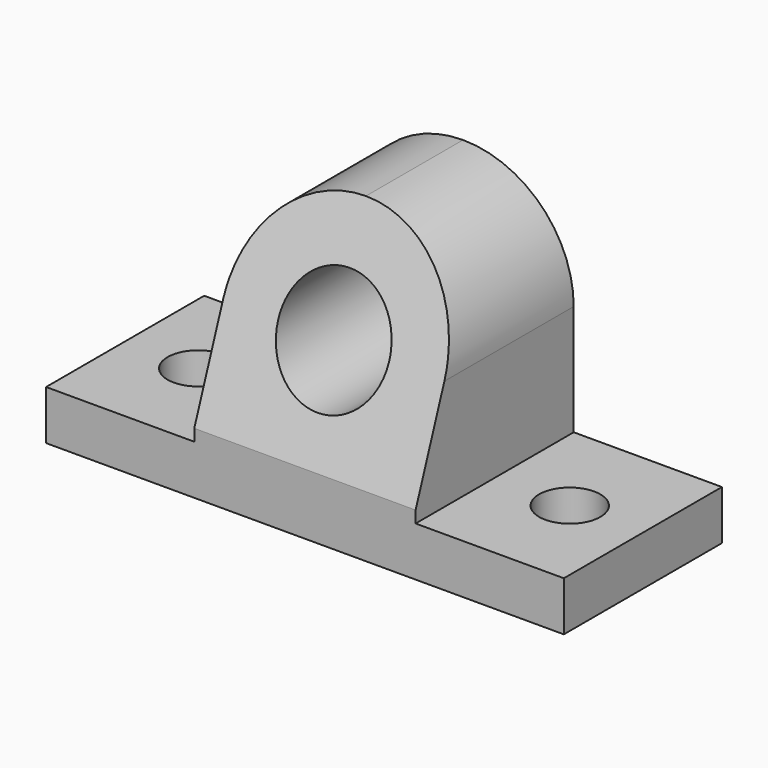
from build123d import *

# Parameters (mm, degrees)
F0_W     = 50.8
F0_H     = 12.7
F0_H_2   = 3.048
F1_DEPTH = 56.896
F2_DEPTH = 94.996
F3_DEPTH = 38.1
F4_R     = 28.44799
F6_DEPTH = 51.054
F8_DEPTH = 42.418


# Not quite as in the source:
# - a fillet or chamfer is up to 0.001 mm smaller than in the source, because OpenCascade refuses the exact size


with BuildPart() as f1:
    # F0 (on Right) → F1 (new body)
    with BuildSketch(Plane.YZ):
        with Locations((25.4, 6.35)):
            Rectangle(F0_W, F0_H)
        Polygon((19.5990691748, 69.596), (0, 15.748), (50.8, 15.748), (50.8, 69.596), align=None)
        with Locations((25.4, 14.224)):
            Rectangle(F0_W, F0_H_2)
    extrude(amount=F1_DEPTH)

    # F0 (on Right) → F2 (join)
    with BuildSketch(Plane.YZ):
        with Locations((25.4, 6.35)):
            Rectangle(F0_W, F0_H)
    extrude(amount=F2_DEPTH)

    # F0 (on Right) → F3 (join)
    with BuildSketch(Plane.YZ):
        with Locations((25.4, 6.35)):
            Rectangle(F0_W, F0_H)
    extrude(amount=-F3_DEPTH)

    # F4 (radius 28.448 in the source; OpenCascade refuses exactly that, so slightly less here)
    f4_edges = [f1.edges().sort_by_distance(p)[0] for p in [
        (0, 35.199535, 69.596),
        (56.896, 35.199535, 69.596),
    ]]
    fillet(f4_edges, radius=F4_R)

    # F5 (on face) → F6 (cut)
    with BuildSketch(Plane(origin=(0, 50.8, 0), x_dir=(-1, 0, 0), z_dir=(0, 1, 0))):
        with BuildLine():
            ThreePointArc((-14.1605, 41.148), (-28.448, 55.4355), (-42.7355, 41.148))
            Line((-42.7355, 41.148), (-14.1605, 41.148))
        make_face()
        with BuildLine():
            Line((-14.1605, 41.148), (-42.7355, 41.148))
            ThreePointArc((-42.7355, 41.148), (-28.448, 26.8605), (-14.1605, 41.148))
        make_face()
    extrude(amount=-F6_DEPTH, mode=Mode.SUBTRACT)

    # F7 (on face) → F8 (cut)
    with BuildSketch(Plane(origin=(0, 0, 0), x_dir=(1, 0, 0), z_dir=(0, 0, -1))):
        with BuildLine():
            ThreePointArc((-11.43, -25.4), (-19.304, -17.526), (-27.178, -25.4))
            Line((-27.178, -25.4), (-19.304, -25.4))
            Line((-19.304, -25.4), (-11.43, -25.4))
        make_face()
        with BuildLine():
            ThreePointArc((84.074, -25.4), (76.2, -17.526), (68.326, -25.4))
            Line((68.326, -25.4), (76.2, -25.4))
            Line((76.2, -25.4), (84.074, -25.4))
        make_face()
        with BuildLine():
            Line((76.2, -25.4), (68.326, -25.4))
            ThreePointArc((68.326, -25.4), (76.2, -33.274), (84.074, -25.4))
            Line((84.074, -25.4), (76.2, -25.4))
        make_face()
        with BuildLine():
            Line((-19.304, -25.4), (-27.178, -25.4))
            ThreePointArc((-27.178, -25.4), (-19.304, -33.274), (-11.43, -25.4))
            Line((-11.43, -25.4), (-19.304, -25.4))
        make_face()
    extrude(amount=-F8_DEPTH, mode=Mode.SUBTRACT)


solid = f1.part
